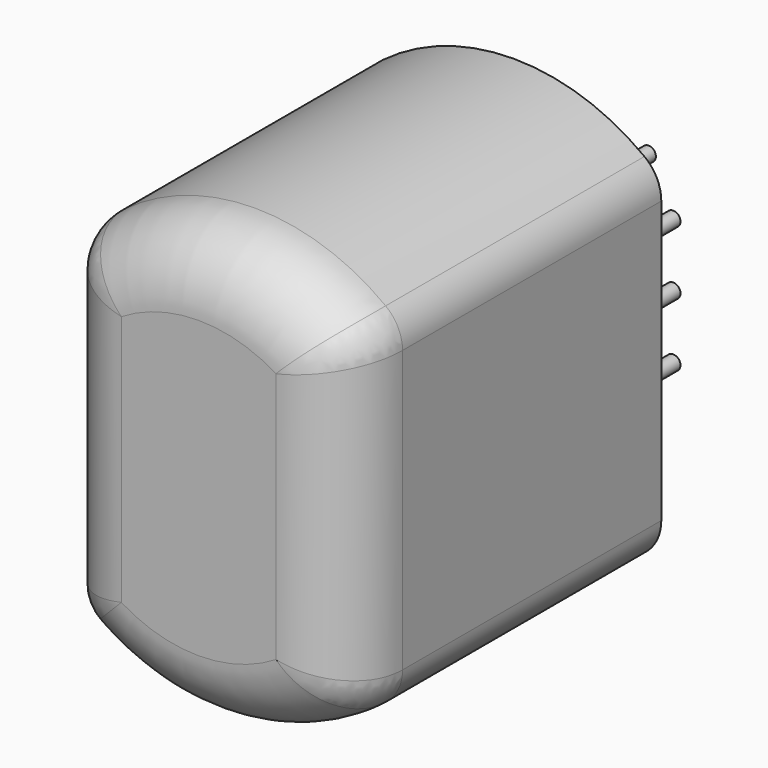
from build123d import *

# Parameters (mm, degrees)
F1_DEPTH    = 28
F2_R        = 0.515
F3_DEPTH    = 7
F4_T1_DEPTH = 47.803508502
F4_T4_ANGLE = 177.7305014171
F4_T6_ANGLE = 177.7305014171
F5_R        = 3


# Not quite as in the source:
# - a fillet or chamfer that OpenCascade refuses, or shapes differently, is made with other operations: its cross-section is extruded or revolved along the edge and cut away or added


with BuildPart() as f1:
    # F0 (on Front) → F1 (new body)
    with BuildSketch(Plane.XZ):
        with BuildLine():
            Line((-10.5, 11.401754251), (-10.5, 0))
            Line((-10.5, 0), (-10.5, -11.401754251))
            ThreePointArc((-10.5, -11.401754251), (0, -15.5), (10.5, -11.401754251))
            Line((10.5, -11.401754251), (10.5, 0))
            Line((10.5, 0), (10.5, 11.401754251))
            ThreePointArc((10.5, 11.401754251), (0, 15.5), (-10.5, 11.401754251))
        make_face()
    extrude(amount=F1_DEPTH)

    # F2 (on face) → F3 (join)
    with BuildSketch(Plane(origin=(0, 0, 0), x_dir=(-1, 0, 0), z_dir=(0, 1, 0))):
        with Locations((-4, 8)):
            Circle(F2_R)
        with Locations((0, 9)):
            Circle(F2_R)
        with Locations((4, 8)):
            Circle(F2_R)
        with Locations((5.75, 4.5)):
            Circle(F2_R)
        with Locations((5.75, 0)):
            Circle(F2_R)
        with Locations((5.75, -4.5)):
            Circle(F2_R)
        with Locations((4, -8)):
            Circle(F2_R)
        with Locations((0, -9)):
            Circle(F2_R)
        with Locations((-4, -8)):
            Circle(F2_R)
        with Locations((-5.75, -4.5)):
            Circle(F2_R)
        with Locations((-5.75, 0)):
            Circle(F2_R)
        with Locations((-5.75, 4.5)):
            Circle(F2_R)
    extrude(amount=F3_DEPTH)

    # F4: fillet of radius 5 on 4 edges, made by hand

    # F4_s2 → F4_t1 (cut)
    with BuildSketch(Plane.XY.offset(-23.901754251)):
        with BuildLine():
            ThreePointArc((-10.5, -23), (-9.0355339059, -26.5355339059), (-5.5, -28))
            Line((-5.5, -28), (-10.5, -28))
            Line((-10.5, -28), (-10.5, -23))
        make_face()
        with BuildLine():
            ThreePointArc((5.5, -28), (9.0355339059, -26.5355339059), (10.5, -23))
            Line((10.5, -23), (10.5, -28))
            Line((10.5, -28), (5.5, -28))
        make_face()
    extrude(amount=F4_T1_DEPTH, mode=Mode.SUBTRACT)

    # F4_s3 → F4_t4 (revolve, cut)
    with BuildSketch(Plane(origin=(0, 0, 0), x_dir=(0, 1, 0), z_dir=(-0.0198038166, 0, 0.9998038852))):
        with BuildLine():
            ThreePointArc((-28, 10.5), (-26.5355339059, 14.0355339059), (-23, 15.5))
            Line((-23, 15.5), (-28, 15.5))
            Line((-28, 15.5), (-28, 10.5))
        make_face()
    revolve(axis=Axis((0, -28, 0), (0, -1, 0)), revolution_arc=F4_T4_ANGLE, mode=Mode.SUBTRACT)

    # F4_s5 → F4_t6 (revolve, cut)
    with BuildSketch(Plane(origin=(0, 0, 0), x_dir=(0, 1, 0), z_dir=(0.0198038166, 0, -0.9998038852))):
        with BuildLine():
            ThreePointArc((-23, 15.5), (-26.5355339059, 14.0355339059), (-28, 10.5))
            Line((-28, 10.5), (-28, 15.5))
            Line((-28, 15.5), (-23, 15.5))
        make_face()
    revolve(axis=Axis((0, -28, 0), (0, -1, 0)), revolution_arc=F4_T6_ANGLE, mode=Mode.SUBTRACT)

    # F5
    f5_edges = [f1.edges().sort_by_distance(p)[0] for p in [
        (8.924732, -26.642967, 10.688654),
        (-8.924732, -26.642967, 10.688654),
        (-8.924732, -26.642967, -10.688654),
        (8.924732, -26.642967, -10.688654),
        (-10.5, -11.5, -11.401754),
        (-10.5, -11.5, 11.401754),
        (10.5, -11.5, -11.401754),
        (10.5, -11.5, 11.401754),
    ]]
    fillet(f5_edges, radius=F5_R)


solid = f1.part
